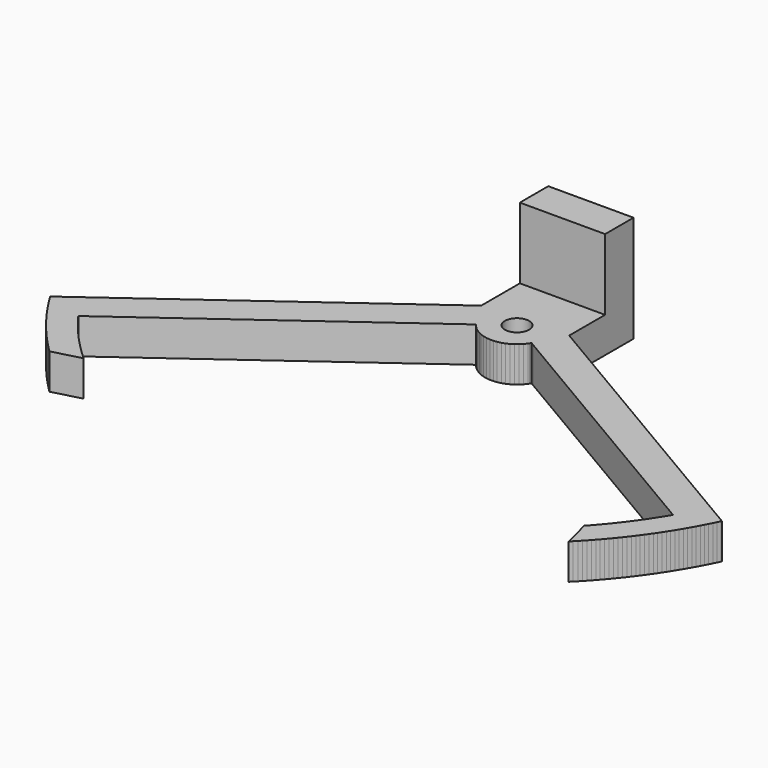
from build123d import *

# Parameters (mm, degrees)
F0_R     = 1.7
F1_DEPTH = 5
F0_W     = 4.5
F0_H     = 5
F0_W_2   = 3
F2_DEPTH = 15


# Not quite as in the source:
# - a feature names something its author has since deleted; it is built from what else it names


with BuildPart() as f1:
    # F0 (on Top) → F1 (new body)
    with BuildSketch(Plane.XY):
        with BuildLine():
            Line((-37.42359, -20.713661), (-33.444589, -19.664665))
            Line((-33.444589, -19.664665), (-33.814619, -19.328399))
            Line((-33.814619, -19.328399), (-34.181145, -18.988316))
            Line((-34.181145, -18.988316), (-34.544128, -18.644454))
            Line((-34.544128, -18.644454), (-34.903529, -18.29685))
            Line((-34.903529, -18.29685), (-35.259309, -17.94554))
            Line((-35.259309, -17.94554), (-35.611429, -17.590562))
            Line((-35.611429, -17.590562), (-35.959853, -17.231955))
            Line((-35.959853, -17.231955), (-36.304542, -16.869758))
            Line((-36.304542, -16.869758), (-36.645459, -16.504008))
            Line((-36.645459, -16.504008), (-36.982569, -16.134745))
            Line((-36.982569, -16.134745), (-37.315835, -15.76201))
            Line((-37.315835, -15.76201), (-37.64522, -15.385841))
            Line((-37.64522, -15.385841), (-37.97069, -15.00628))
            Line((-37.97069, -15.00628), (-38.29221, -14.623366))
            Line((-38.29221, -14.623366), (-38.609746, -14.237142))
            Line((-38.609746, -14.237142), (-38.923262, -13.847648))
            Line((-38.923262, -13.847648), (-39.232726, -13.454927))
            Line((-39.232726, -13.454927), (-39.538104, -13.059021))
            Line((-39.538104, -13.059021), (-39.839363, -12.659971))
            Line((-39.839363, -12.659971), (-40.136472, -12.257822))
            Line((-40.136472, -12.257822), (-40.199223, -12.171758))
            Line((-40.199223, -12.171758), (-4.815801, 13.567638))
            Line((-4.815801, 13.567638), (-4.499835, 13.180458))
            Line((-4.499835, 13.180458), (-4.142886, 12.8307))
            Line((-4.142886, 12.8307), (-3.749356, 12.522679))
            Line((-3.749356, 12.522679), (-3.324099, 12.260193))
            Line((-3.324099, 12.260193), (-2.872359, 12.046479))
            Line((-2.872359, 12.046479), (-2.399707, 11.884173))
            Line((-2.399707, 11.884173), (-1.911973, 11.775276))
            Line((-1.911973, 11.775276), (-1.415172, 11.721133))
            Line((-1.415172, 11.721133), (-0.91543, 11.72241))
            Line((-0.91543, 11.72241), (-0.418912, 11.779092))
            Line((-0.418912, 11.779092), (0.068259, 11.890479))
            Line((0.068259, 11.890479), (0.540075, 12.055198))
            Line((0.540075, 12.055198), (0.990717, 12.271218))
            Line((0.990717, 12.271218), (1.414627, 12.535874))
            Line((1.414627, 12.535874), (1.806578, 12.845903))
            Line((1.806578, 12.845903), (2.161735, 13.19748))
            Line((2.161735, 13.19748), (2.475718, 13.58627))
            Line((2.475718, 13.58627), (2.5697381369, 13.7302913689))
            Line((2.5697381369, 13.7302913689), (1.9580461126, 13.7302913689))
            ThreePointArc((1.9580461126, 13.7302913689), (-1.176782, 12.214814), (-4.3116101126, 13.7302913689))
            Line((-4.3116101126, 13.7302913689), (-7.176782, 13.7302913689))
            Line((-7.176782, 13.7302913689), (-7.176782, 17.4148470867))
            Line((-7.176782, 17.4148470867), (-45.510085, -10.470418))
            Line((-45.510085, -10.470418), (-45.250166, -10.897548))
            Line((-45.250166, -10.897548), (-44.986132, -11.322146))
            Line((-44.986132, -11.322146), (-44.718008, -11.744174))
            Line((-44.718008, -11.744174), (-44.445818, -12.163591))
            Line((-44.445818, -12.163591), (-44.169588, -12.580359))
            Line((-44.169588, -12.580359), (-43.889344, -12.994438))
            Line((-43.889344, -12.994438), (-43.605112, -13.405789))
            Line((-43.605112, -13.405789), (-43.316919, -13.814376))
            Line((-43.316919, -13.814376), (-43.024791, -14.220158))
            Line((-43.024791, -14.220158), (-42.728755, -14.623099))
            Line((-42.728755, -14.623099), (-42.428841, -15.02316))
            Line((-42.428841, -15.02316), (-42.125074, -15.420305))
            Line((-42.125074, -15.420305), (-41.817484, -15.814496))
            Line((-41.817484, -15.814496), (-41.5061, -16.205696))
            Line((-41.5061, -16.205696), (-41.19095, -16.59387))
            Line((-41.19095, -16.59387), (-40.872064, -16.97898))
            Line((-40.872064, -16.97898), (-40.549472, -17.360991))
            Line((-40.549472, -17.360991), (-40.223203, -17.739867))
            Line((-40.223203, -17.739867), (-39.893289, -18.115572))
            Line((-39.893289, -18.115572), (-39.55976, -18.488072))
            Line((-39.55976, -18.488072), (-39.222648, -18.857333))
            Line((-39.222648, -18.857333), (-38.881982, -19.223318))
            Line((-38.881982, -19.223318), (-38.537797, -19.585995))
            Line((-38.537797, -19.585995), (-38.190123, -19.945329))
            Line((-38.190123, -19.945329), (-37.838993, -20.301287))
            Line((-37.838993, -20.301287), (-37.484441, -20.653835))
            Line((-37.484441, -20.653835), (-37.42359, -20.713661))
        make_face()
        with BuildLine():
            Line((-3.823958, 19.853833), (-7.176782, 17.4148470867))
            Line((-7.176782, 17.4148470867), (-7.176782, 13.7302913689))
            Line((-7.176782, 13.7302913689), (-4.3116101126, 13.7302913689))
            ThreePointArc((-4.3116101126, 13.7302913689), (-2.4922073209, 19.9923338511), (2.823218, 16.214814))
            ThreePointArc((2.823218, 16.214814), (2.6007378511, 14.8993886791), (1.9580461126, 13.7302913689))
            Line((1.9580461126, 13.7302913689), (2.5697381369, 13.7302913689))
            Line((2.5697381369, 13.7302913689), (2.699204, 13.928609))
            Line((2.699204, 13.928609), (3.0354278194, 13.7302913689))
            Line((3.0354278194, 13.7302913689), (4.823218, 13.7302913689))
            Line((4.823218, 13.7302913689), (4.823218, 17.9002620213))
            Line((4.823218, 17.9002620213), (1.109423, 20.0908))
            Line((1.109423, 20.0908), (0.665545, 20.320399))
            Line((0.665545, 20.320399), (0.198946, 20.499364))
            Line((0.198946, 20.499364), (-0.284619, 20.625488))
            Line((-0.284619, 20.625488), (-0.779188, 20.697215))
            Line((-0.779188, 20.697215), (-1.27866, 20.713661))
            Line((-1.27866, 20.713661), (-1.776876, 20.674622))
            Line((-1.776876, 20.674622), (-2.267691, 20.580581))
            Line((-2.267691, 20.580581), (-2.745051, 20.432696))
            Line((-2.745051, 20.432696), (-3.20307, 20.232793))
            Line((-3.20307, 20.232793), (-3.636099, 19.983336))
            Line((-3.636099, 19.983336), (-3.823958, 19.853833))
        make_face()
        Polygon((4.823218, 13.7302913689), (3.0354278194, 13.7302913689), (40.38674, -8.300937), (40.13049, -8.730279), (39.869806, -9.156942), (39.604715, -9.580881), (39.335246, -10.002051), (39.061427, -10.420406), (38.783288, -10.835901), (38.500859, -11.248493), (38.21417, -11.658135), (37.923252, -12.064786), (37.628136, -12.4684), (37.328853, -12.868934), (37.025437, -13.266346), (36.71792, -13.660593), (36.406334, -14.051633), (36.090712, -14.439423), (35.77109, -14.823922), (35.447501, -15.205088), (35.11998, -15.582882), (34.788562, -15.957261), (34.453283, -16.328186), (34.381366, -16.406751), (35.390903, -20.395946), (35.742952, -20.040897), (36.091554, -19.682463), (36.436676, -19.320678), (36.778286, -18.955574), (37.116352, -18.587187), (37.450843, -18.21555), (37.781727, -17.840698), (38.108974, -17.462667), (38.432553, -17.081492), (38.752433, -16.697207), (39.068585, -16.30985), (39.38098, -15.919456), (39.689588, -15.526061), (39.99438, -15.129703), (40.295328, -14.730418), (40.592404, -14.328244), (40.885581, -13.923219), (41.174829, -13.515379), (41.460124, -13.104763), (41.741437, -12.69141), (42.018744, -12.275358), (42.292017, -11.856646), (42.561231, -11.435313), (42.826362, -11.011398), (43.087385, -10.584942), (43.344274, -10.155983), (43.597007, -9.724561), (43.845559, -9.290718), (44.089907, -8.854494), (44.330029, -8.415928), (44.565902, -7.975063), (44.797505, -7.53194), (45.024814, -7.086599), (45.24781, -6.639083), (45.466471, -6.189433), (45.510086, -6.098405), (4.823218, 17.9002620213), align=None)
        Polygon((-7.176782, 24.214814), (-7.176782, 17.4148470867), (-3.823958, 19.853833), (-3.636099, 19.983336), (-3.20307, 20.232793), (-2.745051, 20.432696), (-2.267691, 20.580581), (-1.776876, 20.674622), (-1.27866, 20.713661), (-0.779188, 20.697215), (-0.284619, 20.625488), (0.198946, 20.499364), (0.665545, 20.320399), (1.109423, 20.0908), (4.823218, 17.9002620213), (4.823218, 24.214814), (0.323218, 24.214814), (-2.676782, 24.214814), align=None)
        with BuildLine():
            ThreePointArc((2.823218, 16.214814), (-2.4922073209, 19.9923338511), (-4.3116101126, 13.7302913689))
            Line((-4.3116101126, 13.7302913689), (1.9580461126, 13.7302913689))
            ThreePointArc((1.9580461126, 13.7302913689), (2.6007378511, 14.8993886791), (2.823218, 16.214814))
        make_face()
        with Locations((-1.176782, 16.214814)):
            Circle(F0_R, mode=Mode.SUBTRACT)
        with BuildLine():
            Line((1.9580461126, 13.7302913689), (-4.3116101126, 13.7302913689))
            ThreePointArc((-4.3116101126, 13.7302913689), (-1.176782, 12.214814), (1.9580461126, 13.7302913689))
        make_face()
    extrude(amount=F1_DEPTH)

    # F0 (on Top) → F2 (join)
    with BuildSketch(Plane.XY):
        with Locations((-4.926782, 26.714814)):
            Rectangle(F0_W, F0_H)
        with Locations((2.573218, 26.714814)):
            Rectangle(F0_W, F0_H)
        with Locations((-1.176782, 26.714814)):
            Rectangle(F0_W_2, F0_H)
    extrude(amount=F2_DEPTH)


solid = f1.part
